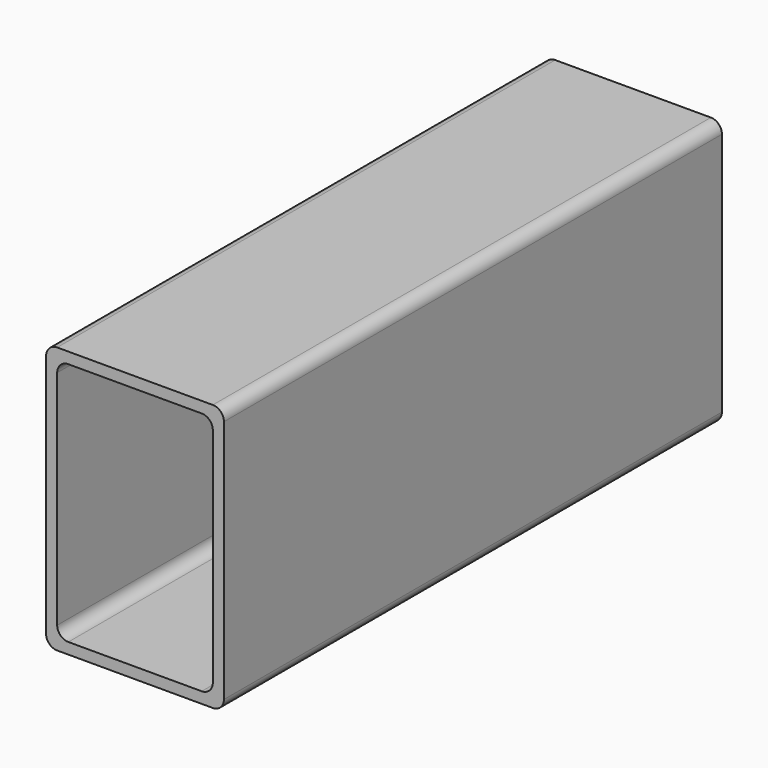
from build123d import *

# Parameters (mm, degrees)
F0_W     = 50.8
F0_H     = 76.2
F0_W_2   = 44.45
F0_H_2   = 69.85
F2_DEPTH = 177.8
F3_R     = 3.175


# Not quite as in the source:
# - a variable given as a bare number and used for a length is read in inches; the dataset says mm whatever the document's units were


with BuildPart() as f2:
    # F0 (on Front) → F2 (new body)
    with BuildSketch(Plane.XZ):
        Rectangle(F0_W, F0_H)
        Rectangle(F0_W_2, F0_H_2, mode=Mode.SUBTRACT)
    extrude(amount=F2_DEPTH)

    # F3
    f3_edges = [f2.edges().sort_by_distance(p)[0] for p in [
        (-22.225, -88.9, 34.925),
        (22.225, -88.9, 34.925),
        (22.225, -88.9, -34.925),
        (-22.225, -88.9, -34.925),
        (25.4, -88.9, 38.1),
        (25.4, -88.9, -38.1),
        (-25.4, -88.9, 38.1),
        (-25.4, -88.9, -38.1),
    ]]
    fillet(f3_edges, radius=F3_R)


solid = f2.part
